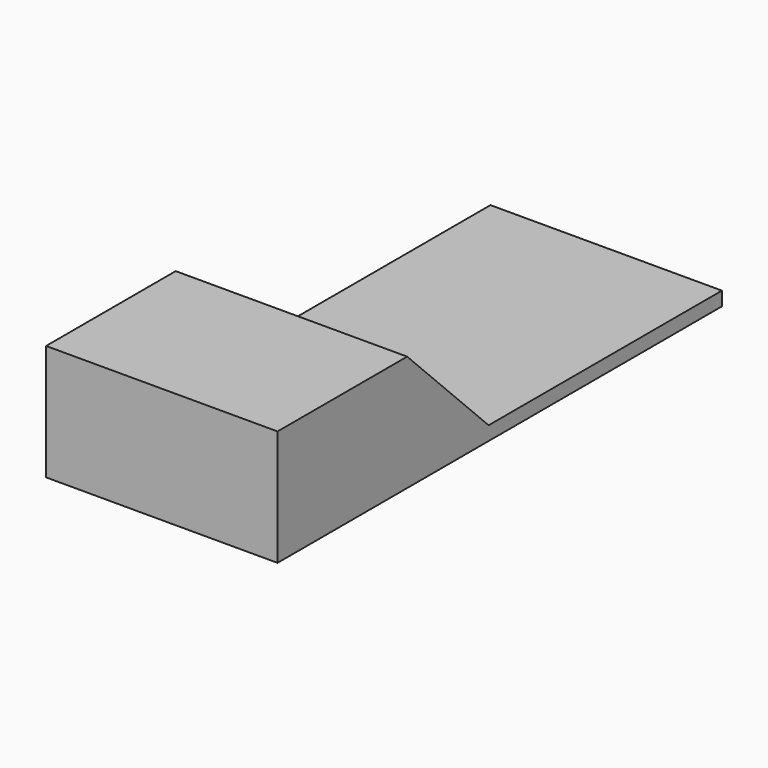
from build123d import *

# Parameters (mm, degrees)
F0_W        = 10
F0_H        = 10
F0_H_2      = 2
F0_H_3      = 12
F1_DEPTH    = 0.6
F2_DEPTH    = 5
F3_T4_DEPTH = 35.7168298797


# Not quite as in the source:
# - a fillet or chamfer that OpenCascade refuses, or shapes differently, is made with other operations: its cross-section is extruded or revolved along the edge and cut away or added


with BuildPart() as f1:
    # F0 (on Top) → F1 (new body)
    with BuildSketch(Plane.XY):
        with Locations((5, 5)):
            Rectangle(F0_W, F0_H)
        with Locations((5, -1)):
            Rectangle(F0_W, F0_H_2)
        with Locations((5, -8)):
            Rectangle(F0_W, F0_H_3)
    extrude(amount=F1_DEPTH)

    # F0 (on Top) → F2 (join)
    with BuildSketch(Plane.XY):
        with Locations((5, -8)):
            Rectangle(F0_W, F0_H_3)
    extrude(amount=F2_DEPTH)

    # F3: chamfer of 5 on 1 edges, made by hand


with BuildPart() as f3_tool2:
    # F3_s3 → F3_t4 (new body)
    with BuildSketch(Plane.YZ.offset(22.8584149398)):
        Polygon((-7, 5), (-2, 0), (-2, 5), align=None)
    extrude(amount=-F3_T4_DEPTH)

    split(bisect_by=Plane.XY.offset(0.6), keep=Keep.TOP)


with BuildPart() as f1_1:
    add(f1.part)

    # F3_t1: cut F3_tool2
    add(f3_tool2.part, mode=Mode.SUBTRACT)


solid = f1_1.part
